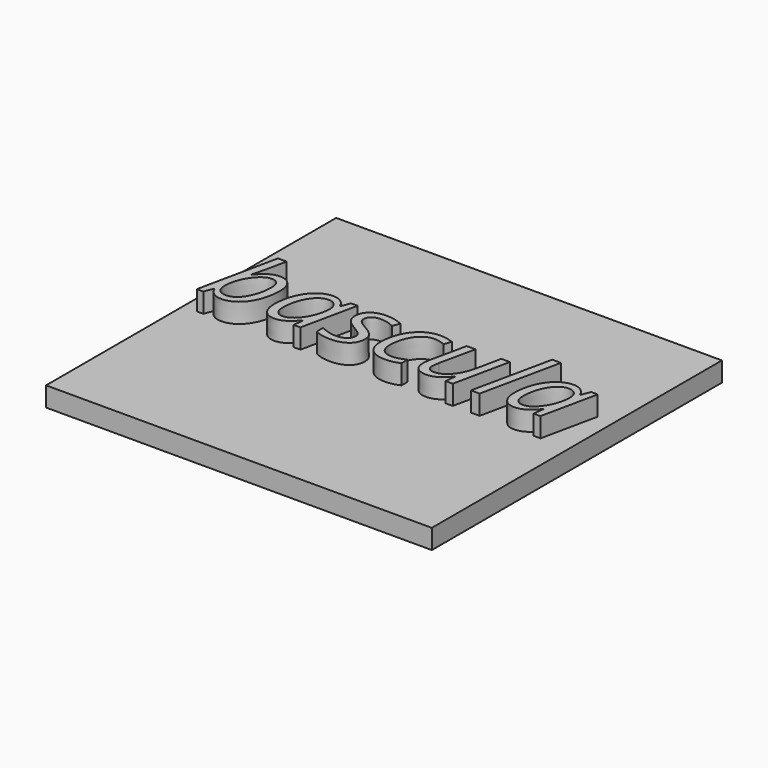
from build123d import *

# Parameters (mm, degrees)
F0_W         = 500
F0_H         = 470
F1_DEPTH     = 25.4
F2_TEXT_SIZE = 136.8218719054
F3_DEPTH     = 25.4


# Not quite as in the source:
# - Text() gives the source's letters only with a copy of the font that has no kerning and outlines rounded to 1/6400 em; it was checked with that copy


with BuildPart() as f1:
    # F0 (on Top) → F1 (new body)
    with BuildSketch(Plane.XY):
        with Locations((-0.8634179831, 150.9907400204)):
            Rectangle(F0_W, F0_H)
    extrude(amount=F1_DEPTH)

    # F2 (on face) → F3 (join)
    with BuildSketch(Plane.XY.offset(25.4)):
        with Locations((-236.9370009886, 137.868060894)):
            Text('bascula', F2_TEXT_SIZE, font='Open Sans', font_style=FontStyle.ITALIC, text_align=(TextAlign.LEFT, TextAlign.BOTTOM))
    extrude(amount=F3_DEPTH)


solid = f1.part
